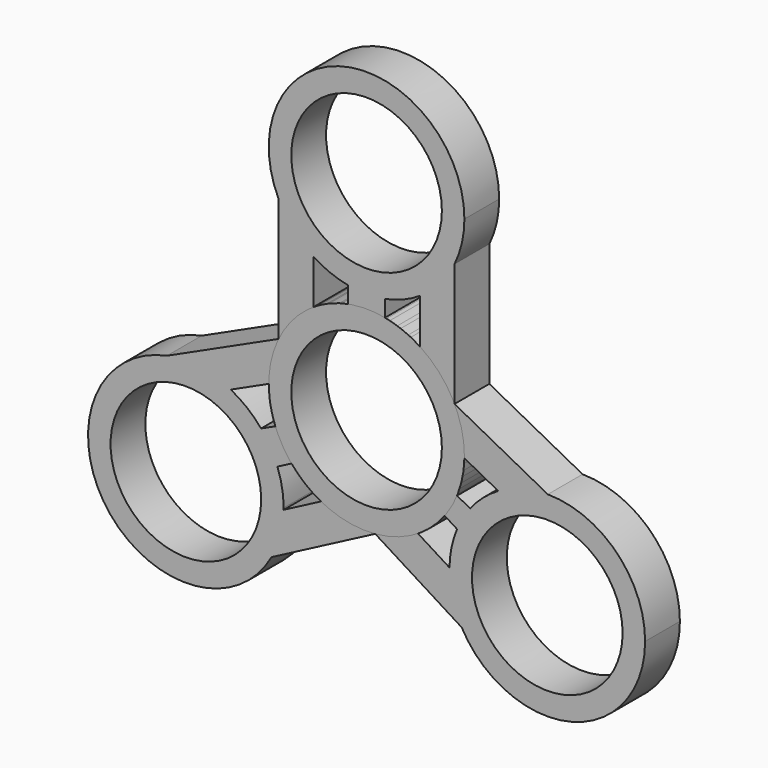
from build123d import *

# Parameters (mm, degrees)
F1_R     = 10.9982
F2_DEPTH = 6.35
F0_R     = 14.2875
F0_R_2   = 10.9982


# Not quite as in the source:
# - a feature names something its author has since deleted; it is built from what else it names


with BuildPart() as f2:
    # F1 (on Front) → F2 (new body)
    with BuildSketch(Plane.XZ):
        with BuildLine():
            ThreePointArc((-19.843860944, -2.5436943773), (-24.3914551143, -1.0938827063), (-29.162820574, -1.2228721227))
            ThreePointArc((-29.162820574, -1.2228721227), (-37.9387049837, -23.660754454), (-13.8928706881, -22.1532519791))
            ThreePointArc((-13.8928706881, -22.1532519791), (-12.5937995119, -18.9304439908), (-12.1111303918, -15.4893529181))
            ThreePointArc((-12.1111303918, -15.4893529181), (-12.1094983388, -15.3646812066), (-12.1089543073, -15.24))
            ThreePointArc((-12.1089543073, -15.24), (-12.3375720505, -12.6943201423), (-13.0161089443, -10.2301083629))
            ThreePointArc((-13.0161089443, -10.2301083629), (-14.0409790879, -8.0653997775), (-15.4130498534, -6.102304292))
            ThreePointArc((-15.4130498534, -6.102304292), (-17.4497380945, -4.100479128), (-19.843860944, -2.5436943773))
        make_face()
        with Locations((-26.3964543073, -15.24)):
            Circle(F1_R, mode=Mode.SUBTRACT)
        with BuildLine():
            ThreePointArc((12.8504353504, 24.2350846639), (13.9235995942, 27.2759353017), (14.2875, 30.48))
            ThreePointArc((14.2875, 30.48), (-3.2040646983, 44.4035995942), (-12.8504353504, 24.2350846639))
            ThreePointArc((-12.8504353504, 24.2350846639), (-10.7030708192, 21.0154909641), (-7.7704353504, 18.4902964709))
            ThreePointArc((-7.7704353504, 18.4902964709), (-5.3291739909, 17.2235841637), (-2.6904353504, 16.4481001331))
            ThreePointArc((-2.6904353504, 16.4481001331), (0, 16.1925), (2.6904353504, 16.4481001331))
            ThreePointArc((2.6904353504, 16.4481001331), (5.3291739909, 17.2235841637), (7.7704353504, 18.4902964709))
            ThreePointArc((7.7704353504, 18.4902964709), (10.7030708192, 21.0154909641), (12.8504353504, 24.2350846639))
        make_face()
        with Locations((0, 30.48)):
            Circle(F1_R, mode=Mode.SUBTRACT)
        with BuildLine():
            ThreePointArc((40.6839543073, -15.24), (36.5249191169, -5.162953962), (26.4691711959, -0.9526850492))
            ThreePointArc((26.4691711959, -0.9526850492), (22.7246778763, -1.4323675422), (19.2365261049, -2.8760166457))
            ThreePointArc((19.2365261049, -2.8760166457), (17.011936244, -4.4667239445), (15.1311826772, -6.452149788))
            ThreePointArc((15.1311826772, -6.452149788), (14.0619860916, -8.0293446841), (13.2121716662, -9.7347890605))
            ThreePointArc((13.2121716662, -9.7347890605), (12.4074813108, -12.3346100515), (12.1103563293, -15.039848026))
            ThreePointArc((12.1103563293, -15.039848026), (12.5374540198, -18.7128615405), (13.8928706881, -22.1532519791))
            ThreePointArc((13.8928706881, -22.1532519791), (29.9663076159, -29.0743342306), (40.6839543073, -15.24))
        make_face()
        with Locations((26.3964543073, -15.24)):
            Circle(F1_R, mode=Mode.SUBTRACT)
        with BuildLine():
            ThreePointArc((-7.7704353504, 11.9897035291), (-10.7030708192, 9.4645090359), (-12.8504353504, 6.2449153361))
            ThreePointArc((-12.8504353504, 6.2449153361), (-13.9235995942, 3.2040646983), (-14.2875, 0))
            ThreePointArc((-14.2875, 0), (-14.0455567318, -2.6182040304), (-13.3279210191, -5.1477351873))
            ThreePointArc((-13.3279210191, -5.1477351873), (-12.3114587928, -7.2498716295), (-10.9661701776, -9.1583714647))
            ThreePointArc((-10.9661701776, -9.1583714647), (-8.9837608827, -11.109666811), (-6.6608286535, -12.6398583021))
            ThreePointArc((-6.6608286535, -12.6398583021), (-2.8160957214, -14.0072217494), (1.2583537723, -14.231978149))
            ThreePointArc((1.2583537723, -14.231978149), (4.5050529518, -13.5586560599), (7.5091136575, -12.1550758257))
            ThreePointArc((7.5091136575, -12.1550758257), (9.623374139, -10.5604605218), (11.4070274702, -8.6030448415))
            ThreePointArc((11.4070274702, -8.6030448415), (12.4109111642, -7.0782724111), (13.2121716662, -5.4379385904))
            ThreePointArc((13.2121716662, -5.4379385904), (13.9903735339, -2.8986384098), (14.2851490362, -0.2591780564))
            ThreePointArc((14.2851490362, -0.2591780564), (14.2869122469, -0.1295943594), (14.2875, 0))
            ThreePointArc((14.2875, 0), (13.9235995942, 3.2040646983), (12.8504353504, 6.2449153361))
            ThreePointArc((12.8504353504, 6.2449153361), (10.7030708192, 9.4645090359), (7.7704353504, 11.9897035291))
            ThreePointArc((7.7704353504, 11.9897035291), (5.3291739909, 13.2564158363), (2.6904353504, 14.0318998669))
            ThreePointArc((2.6904353504, 14.0318998669), (0, 14.2875), (-2.6904353504, 14.0318998669))
            ThreePointArc((-2.6904353504, 14.0318998669), (-5.3291739909, 13.2564158363), (-7.7704353504, 11.9897035291))
        make_face()
        Circle(F1_R, mode=Mode.SUBTRACT)
        with BuildLine():
            ThreePointArc((-7.7704353504, 18.4902964709), (-10.7030708192, 21.0154909641), (-12.8504353504, 24.2350846639))
            Line((-12.8504353504, 24.2350846639), (-12.8504353504, 6.2449153361))
            ThreePointArc((-12.8504353504, 6.2449153361), (-10.7030708192, 9.4645090359), (-7.7704353504, 11.9897035291))
            Line((-7.7704353504, 11.9897035291), (-7.7704353504, 18.4902964709))
        make_face()
        with BuildLine():
            Line((12.8504353504, 6.2449153361), (12.8504353504, 24.2350846639))
            ThreePointArc((12.8504353504, 24.2350846639), (10.7030708192, 21.0154909641), (7.7704353504, 18.4902964709))
            Line((7.7704353504, 18.4902964709), (7.7704353504, 11.9897035291))
            ThreePointArc((7.7704353504, 11.9897035291), (10.7030708192, 9.4645090359), (12.8504353504, 6.2449153361))
        make_face()
        with BuildLine():
            ThreePointArc((7.5091136575, -12.1550758257), (4.5050529518, -13.5586560599), (1.2583537723, -14.231978149))
            Line((1.2583537723, -14.231978149), (13.8928706881, -22.1532519791))
            ThreePointArc((13.8928706881, -22.1532519791), (12.5374540198, -18.7128615405), (12.1103563293, -15.039848026))
            Line((12.1103563293, -15.039848026), (7.5091136575, -12.1550758257))
        make_face()
        with BuildLine():
            ThreePointArc((-12.1111303918, -15.4893529181), (-12.5937995119, -18.9304439908), (-13.8928706881, -22.1532519791))
            Line((-13.8928706881, -22.1532519791), (1.2583537723, -14.231978149))
            ThreePointArc((1.2583537723, -14.231978149), (-2.8160957214, -14.0072217494), (-6.6608286535, -12.6398583021))
            Line((-6.6608286535, -12.6398583021), (-12.1111303918, -15.4893529181))
        make_face()
        with BuildLine():
            ThreePointArc((-14.2875, 0), (-13.9235995942, 3.2040646983), (-12.8504353504, 6.2449153361))
            Line((-12.8504353504, 6.2449153361), (-29.162820574, -1.2228721227))
            ThreePointArc((-29.162820574, -1.2228721227), (-24.3914551143, -1.0938827063), (-19.843860944, -2.5436943773))
            Line((-19.843860944, -2.5436943773), (-14.2875, 0))
        make_face()
        with BuildLine():
            ThreePointArc((-10.9661701776, -9.1583714647), (-12.3114587928, -7.2498716295), (-13.3279210191, -5.1477351873))
            Line((-13.3279210191, -5.1477351873), (-15.4130498534, -6.102304292))
            ThreePointArc((-15.4130498534, -6.102304292), (-14.0409790879, -8.0653997775), (-13.0161089443, -10.2301083629))
            Line((-13.0161089443, -10.2301083629), (-10.9661701776, -9.1583714647))
        make_face()
        with BuildLine():
            ThreePointArc((2.6904353504, 16.4481001331), (0, 16.1925), (-2.6904353504, 16.4481001331))
            Line((-2.6904353504, 16.4481001331), (-2.6904353504, 14.0318998669))
            ThreePointArc((-2.6904353504, 14.0318998669), (0, 14.2875), (2.6904353504, 14.0318998669))
            Line((2.6904353504, 14.0318998669), (2.6904353504, 16.4481001331))
        make_face()
        with BuildLine():
            Line((26.4691711959, -0.9526850492), (12.8504353504, 6.2449153361))
            ThreePointArc((12.8504353504, 6.2449153361), (13.9235995942, 3.2040646983), (14.2875, 0))
            ThreePointArc((14.2875, 0), (14.2869122469, -0.1295943594), (14.2851490362, -0.2591780564))
            Line((14.2851490362, -0.2591780564), (19.2365261049, -2.8760166457))
            ThreePointArc((19.2365261049, -2.8760166457), (22.7246778763, -1.4323675422), (26.4691711959, -0.9526850492))
        make_face()
        with BuildLine():
            Line((15.1311826772, -6.452149788), (13.2121716662, -5.4379385904))
            ThreePointArc((13.2121716662, -5.4379385904), (12.4109111642, -7.0782724111), (11.4070274702, -8.6030448415))
            Line((11.4070274702, -8.6030448415), (13.2121716662, -9.7347890605))
            ThreePointArc((13.2121716662, -9.7347890605), (14.0619860916, -8.0293446841), (15.1311826772, -6.452149788))
        make_face()
    extrude(amount=F2_DEPTH)


with BuildPart() as f2b:
    # F0 (on Front) → F2, piece 2 (new body)
    with BuildSketch(Plane.XZ):
        Circle(F0_R)
        Circle(F0_R_2, mode=Mode.SUBTRACT)
    extrude(amount=F2_DEPTH)


solid = Compound([f2.part, f2b.part])
